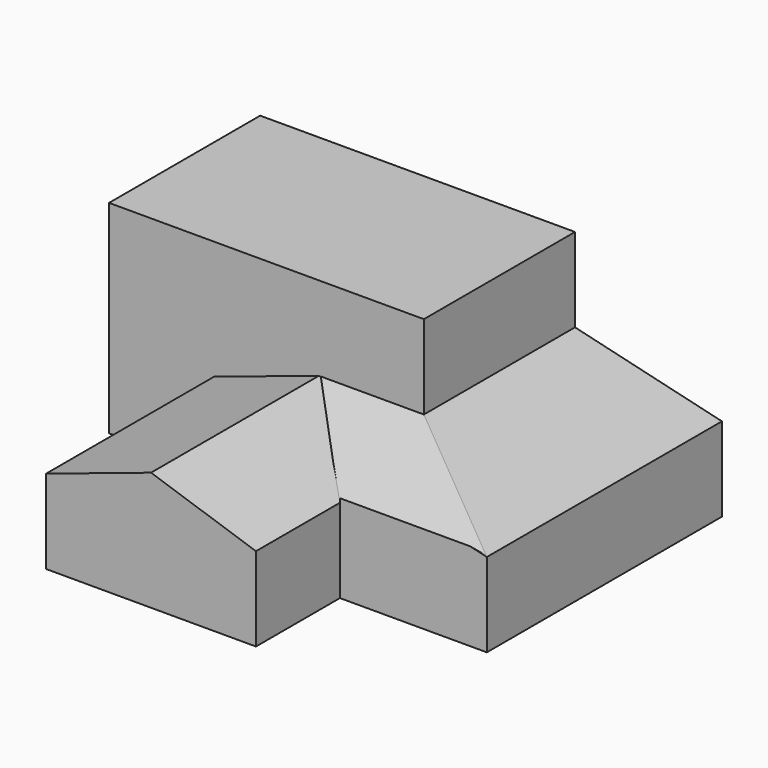
from build123d import *

# Parameters (mm, degrees)
F0_W      = 4267.2
F0_H      = 8534.4
F1_DEPTH  = 3454.4
F3_DEPTH  = 12247.14028
F4_W      = 5486.4
F4_H      = 3454.4
F5_DEPTH  = 9144
F6_DEPTH  = 2438.4
F8_W      = 6096
F8_H      = 3454.4
F9_DEPTH  = 6096
F11_DEPTH = 6096
F13_DEPTH = 6096
F16_DEPTH = 25.4
F18_DEPTH = 3511.20794


with BuildPart() as f1:
    # F0 (on Top) → F1 (new body)
    with BuildSketch(Plane.XY):
        with Locations((2133.6, 4267.2)):
            Rectangle(F0_W, F0_H)
    extrude(amount=F1_DEPTH)

    # F2 (on face) → F3 (cut)
    with BuildSketch(Plane.XZ):
        Polygon((0, 3454.4), (4267.2, 2438.4), (4267.2, 3454.4), align=None)
    extrude(amount=-F3_DEPTH, mode=Mode.SUBTRACT)

    # F4 (on face) → F5 (join)
    with BuildSketch(Plane(origin=(0, 0, 0), x_dir=(0, -1, 0), z_dir=(-1, 0, 0))):
        with Locations((-5791.2, 1727.2)):
            Rectangle(F4_W, F4_H)
    extrude(amount=F5_DEPTH)

    # F6 (add): a face of the model
    f6_faces = [f1.faces().sort_by_distance(p)[0] for p in [
        (-4572, 5791.2, 3454.4),
    ]]
    extrude(f6_faces, amount=F6_DEPTH)

    # F8 (on face) → F9 (join)
    with BuildSketch(Plane.XZ.offset(-3048)):
        with Locations((-3048, 1727.2)):
            Rectangle(F8_W, F8_H)
    extrude(amount=F9_DEPTH)

    # F10 (on face) → F11 (cut)
    with BuildSketch(Plane.XZ.offset(3048)):
        Polygon((-6096, 3454.4), (-6096, 2438.4), (-3048, 3454.4), align=None)
    extrude(amount=-F11_DEPTH, mode=Mode.SUBTRACT)

    # F12 (on face) → F13 (cut)
    with BuildSketch(Plane.XZ.offset(3048)):
        Polygon((0, 3454.4), (-3048, 3454.4), (0, 2438.4), align=None)
    extrude(amount=-F13_DEPTH, mode=Mode.SUBTRACT)

    # F15 (on 3pt) → F16 (join)
    with BuildSketch(Plane(origin=(0, -731.52, 2194.56), x_dir=(1, 0, 0), z_dir=(0, -0.316227766, 0.9486832981))):
        Polygon((-2998.1036186218, 3988.1196022034), (0, 743.2488799095), (0, 3988.1196022034), align=None)
    extrude(amount=-F16_DEPTH)

    # F17 (on 3pt) → F18 (cut)
    with BuildSketch(Plane(origin=(0, -731.52, 2194.56), x_dir=(1, 0, 0), z_dir=(0, -0.316227766, 0.9486832981))):
        Polygon((0, 3984.4744205475), (0, 807.7730536461), (4260.7135772705, 807.7730536461), align=None)
    extrude(amount=F18_DEPTH, mode=Mode.SUBTRACT)


solid = f1.part
